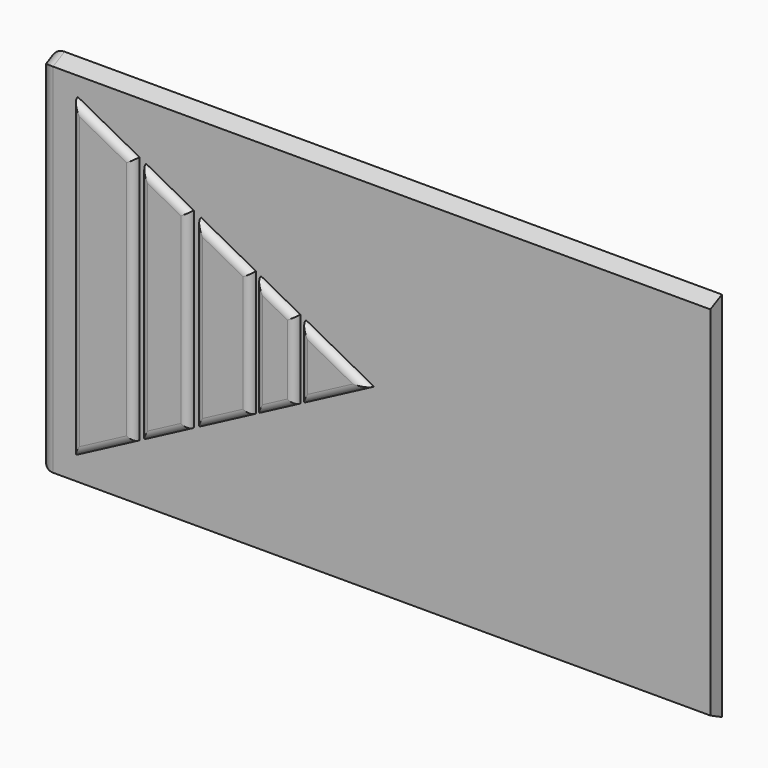
from build123d import *

# Parameters (mm, degrees)
F1_DEPTH       = 93
F2_R           = 1.99999
F4_DEPTH       = 1
F5_R           = 0.99999
F6_ANGLE       = 90
F7_ANGLE       = 90
F8_TEXT_SIZE   = 25.7223611698
F8_TEXT_SIZE_2 = 12.3619506431
F9_DEPTH       = 1


# Not quite as in the source:
# - a fillet or chamfer is up to 0.001 mm smaller than in the source, because OpenCascade refuses the exact size
# - Text() gives the source's letters only with a copy of the font that has no kerning and outlines rounded to 1/6400 em; it was checked with that copy


with BuildPart() as f1:
    # F0 (on Front) → F1 (new body)
    with BuildSketch(Plane.XZ):
        Polygon((-24.75, 1), (-25.75, -1), (25.75, -1), (24.75, 1), align=None)
    extrude(amount=F1_DEPTH)

    # F2 (radius 2 in the source; OpenCascade refuses exactly that, so slightly less here)
    f2_edges = [f1.edges().sort_by_distance(p)[0] for p in [
        (0, -93, 1),
        (25.25, -93, 0),
        (-25.25, -93, 0),
    ]]
    fillet(f2_edges, radius=F2_R)

    # F3 (on face) → F4 (join)
    with BuildSketch(Plane.XY.offset(1)):
        Polygon((4.7301794979, -55.9521774143), (-0.2081218514, -46.5794830167), (-5.2301794979, -55.9521774143), align=None)
        Polygon((-5.6653136183, -56.7642706677), (-8.5675057218, -62.1806480939), (8.0118468452, -62.1806480939), (5.1580565883, -56.7642706677), align=None)
        Polygon((-8.9481600436, -62.891065393), (-13.0165527666, -70.4839295868), (12.3866940833, -70.4839295868), (8.386152734, -62.891065393), align=None)
        Polygon((-13.5663655681, -71.5100483067), (-17.0923142089, -78.0905460626), (16.3944812588, -78.0905460626), (12.9273372799, -71.5100483067), align=None)
        Polygon((-17.6011467683, -79.0401831266), (-22.1620798013, -87.5522780677), (21.3796948959, -87.5522780677), (16.8948276688, -79.0401831266), align=None)
    extrude(amount=F4_DEPTH)

    # F5 (radius 1 in the source; OpenCascade refuses exactly that, so slightly less here)
    f5_edges = [f1.edges().sort_by_distance(p)[0] for p in [
        (-0.25, -55.952177, 2),
        (2.261029, -51.26583, 2),
        (-2.719151, -51.26583, 2),
        (-7.11641, -59.472459, 2),
        (-0.277829, -62.180648, 2),
        (6.584952, -59.472459, 2),
        (-0.253629, -56.764271, 2),
        (-10.982356, -66.687497, 2),
        (-0.314929, -70.48393, 2),
        (10.386423, -66.687497, 2),
        (-0.281004, -62.891065, 2),
        (-19.881613, -83.296231, 2),
        (-0.391192, -87.552278, 2),
        (19.137261, -83.296231, 2),
        (-0.35316, -79.040183, 2),
        (-0.319514, -71.510048, 2),
        (-15.32934, -74.800297, 2),
        (-0.348916, -78.090546, 2),
        (14.660909, -74.800297, 2),
    ]]
    fillet(f5_edges, radius=F5_R)


with BuildPart() as f1_1:
    # F6: moved
    add(f1.part.rotate(Axis((-25.75, -46.5, -1), (0, 1, 0)), F6_ANGLE))


with BuildPart() as f1_2:
    # F7: moved
    add(f1_1.part.rotate(Axis((-23.75, 0, -26.75), (0, 0, -1)), F7_ANGLE))

    # F8 (on face) → F9 (cut)
    with BuildSketch(Plane(origin=(0, 2, 0), x_dir=(-1, 0, 0), z_dir=(0, 1, 0))):
        with Locations((34.0922623873, -43.0316217244)):
            Text('Diana', F8_TEXT_SIZE, font='Open Sans', font_style=FontStyle.BOLD, text_align=(TextAlign.LEFT, TextAlign.BOTTOM))
        with Locations((28.4477278257, -15.4894103076)):
            Text('Propiedad de:', F8_TEXT_SIZE_2, font='Open Sans', font_style=FontStyle.BOLD, text_align=(TextAlign.LEFT, TextAlign.BOTTOM))
    extrude(amount=-F9_DEPTH, mode=Mode.SUBTRACT)


solid = f1_2.part
